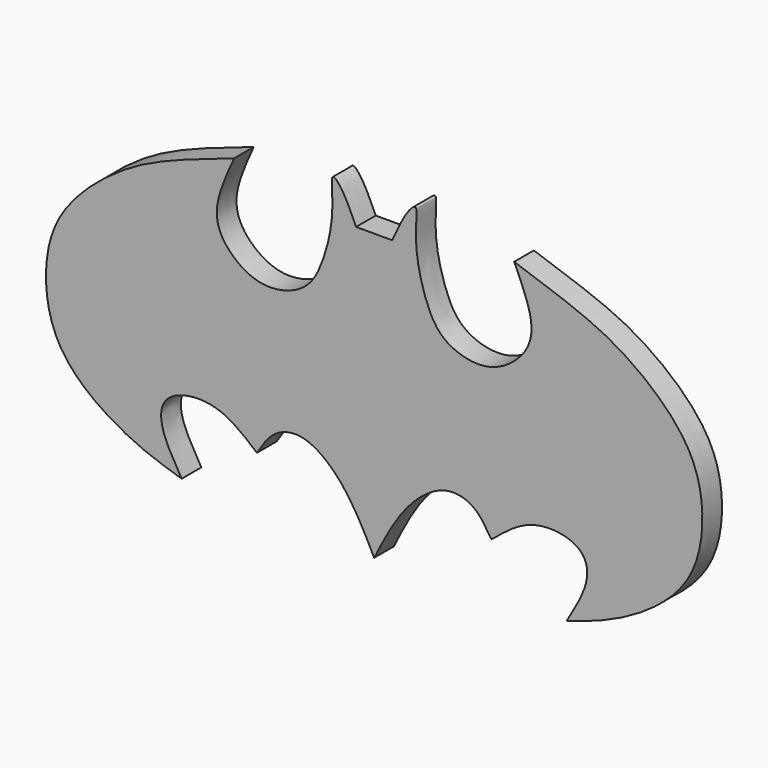
from build123d import *

# Parameters (mm, degrees)
F1_DEPTH = 5


with BuildPart() as f1:
    # F0 (on Front) → F1 (new body)
    with BuildSketch(Plane.XZ):
        with BuildLine():
            Line((-8.2122022286, 40.0784350932), (-11.8819409981, 40.0784350932))
            add(Edge.make_bspline(
                [(-11.8819409981, 40.0784350932), (-12.8782472371, 42.2972484802), (-14.4335544357, 45.7609791067), (-17.3519257227, 48.7913666131), (-16.0950854738, 41.2351091341), (-18.4014485043, 31.4854467346), (-22.0437905993, 24.85808478), (-31.2282103596, 22.4385748293), (-38.4247454255, 27.2876434832), (-41.4317275403, 33.8661623662), (-38.41791048, 40.5091837611), (-36.6988517344, 44.2983135581)],
                knots=[0, 0, 0, 0, 0.1088146702, 0.1698676905, 0.2662726076, 0.4039159487, 0.5157076846, 0.6364836069, 0.7547343235, 0.8601022896, 1, 1, 1, 1], degree=3))
            add(Edge.make_bspline(
                [(-36.6988517344, 44.2983135581), (-40.7675535004, 42.9207700785), (-48.8190673042, 40.1947628707), (-59.720474171, 35.363141512), (-72.7769239422, 24.2824619419), (-75.9139064544, 11.2929836241), (-73.1167440149, -3.1146307179), (-58.8360799137, -12.9740366543), (-50.9861442753, -15.4269461348), (-47.3704449832, -16.5567621589)],
                knots=[0, 0, 0, 0, 0.1374294184, 0.271957721, 0.4283369128, 0.5665488064, 0.709317309, 0.8661108513, 1, 1, 1, 1], degree=3))
            add(Edge.make_bspline(
                [(-47.3704449832, -16.5567621589), (-49.0258540698, -13.767318885), (-51.8526301052, -9.0040664284), (-51.5200005236, -3.7669274307), (-47.3638537079, -1.00085823), (-39.2892684136, -0.8731954731), (-34.5610362718, -4.8462458488), (-32.0631302893, -6.9451923482)],
                knots=[0, 0, 0, 0, 0.2300305605, 0.3928001127, 0.553391391, 0.764058472, 1, 1, 1, 1], degree=3))
            add(Edge.make_bspline(
                [(-32.0631302893, -6.9451923482), (-30.9825657831, -5.1874304781), (-28.8354937584, -1.6947733382), (-22.0931432409, -0.1443481526), (-13.8550388164, -6.7624223585), (-10.1796756768, -14.0692507531), (-8.2122022286, -17.9806984961)],
                knots=[0, 0, 0, 0, 0.2112971318, 0.419845514, 0.689435165, 1, 1, 1, 1], degree=3))
            add(Edge.make_bspline(
                [(15.6387258321, -6.9451923482), (14.5581613259, -5.1874304781), (12.4110893012, -1.6947733382), (5.6687387837, -0.1443481526), (-2.5693656408, -6.7624223585), (-6.2447287804, -14.0692507531), (-8.2122022286, -17.9806984961)],
                knots=[0, 0, 0, 0, 0.2112971318, 0.419845514, 0.689435165, 1, 1, 1, 1], degree=3))
            add(Edge.make_bspline(
                [(30.946040526, -16.5567621589), (32.6014496126, -13.767318885), (35.428225648, -9.0040664284), (35.0955960664, -3.7669274307), (30.9394492507, -1.00085823), (22.8648639564, -0.8731954731), (18.1366318146, -4.8462458488), (15.6387258321, -6.9451923482)],
                knots=[0, 0, 0, 0, 0.2300305605, 0.3928001127, 0.553391391, 0.764058472, 1, 1, 1, 1], degree=3))
            add(Edge.make_bspline(
                [(20.2744472772, 44.2983135581), (24.3431490432, 42.9207700785), (32.394662847, 40.1947628707), (43.2960697138, 35.363141512), (56.352519485, 24.2824619419), (59.4895019971, 11.2929836241), (56.6923395577, -3.1146307179), (42.4116754565, -12.9740366543), (34.5617398181, -15.4269461348), (30.946040526, -16.5567621589)],
                knots=[0, 0, 0, 0, 0.1374294184, 0.271957721, 0.4283369128, 0.5665488064, 0.709317309, 0.8661108513, 1, 1, 1, 1], degree=3))
            add(Edge.make_bspline(
                [(-4.5424634591, 40.0784350932), (-3.5461572201, 42.2972484802), (-1.9908500215, 45.7609791067), (0.9275212655, 48.7913666131), (-0.3293189834, 41.2351091341), (1.9770440471, 31.4854467346), (5.6193861421, 24.85808478), (14.8038059024, 22.4385748293), (22.0003409683, 27.2876434832), (25.0073230831, 33.8661623662), (21.9935060227, 40.5091837611), (20.2744472772, 44.2983135581)],
                knots=[0, 0, 0, 0, 0.1088146702, 0.1698676905, 0.2662726076, 0.4039159487, 0.5157076846, 0.6364836069, 0.7547343235, 0.8601022896, 1, 1, 1, 1], degree=3))
            Line((-4.5424634591, 40.0784350932), (-8.2122022286, 40.0784350932))
        make_face()
        with BuildLine():
            add(Edge.make_bspline(
                [(-40.7788082957, 40.8485867083), (-45.0160925485, 39.1557450069), (-53.0935510599, 35.9287114181), (-62.2941692207, 30.6878977022), (-71.2479782326, 20.5851416615), (-73.0395933906, 13.1368363398), (-70.655821628, 0.3918412405), (-65.9333309108, -4.7486149953), (-56.4205247664, -11.0687593178), (-52.9760592159, -12.4550883248), (-51.5802241862, -13.0168842152)],
                knots=[0, 0, 0, 0, 0.1450786062, 0.2765607292, 0.4190573419, 0.5300860887, 0.6687412322, 0.7763945775, 0.9093861509, 1, 1, 1, 1], degree=3))
            add(Edge.make_bspline(
                [(-12.7671184018, 37.1527262032), (-12.8105221655, 37.767832184), (-12.9167695581, 39.2735404689), (-14.2569275875, 43.199559326), (-15.3833842453, 44.8124103405), (-15.4205368039, 43.5883704744), (-15.2325001114, 42.0644743626), (-15.5858480298, 37.7221519204), (-16.6233242245, 33.2855966544), (-18.8663482525, 24.8126850649), (-23.665219481, 22.8462807986), (-32.7768476073, 20.7730831752), (-39.0865075301, 23.8717377388), (-43.0417250552, 31.6481993654), (-41.5266216034, 37.7005347177), (-40.999533454, 39.9194052312), (-40.7788082957, 40.8485867083)],
                knots=[0, 0, 0, 0, 0.0505373663, 0.1237096266, 0.1629392742, 0.1913954138, 0.2358051509, 0.3063180282, 0.384250961, 0.4831926503, 0.5605011807, 0.6644710974, 0.7540445736, 0.853320775, 0.9385761278, 1, 1, 1, 1], degree=3))
            add(Edge.make_bspline(
                [(-3.9949859492, 37.1527262032), (-6.9190301001, 37.1527262032), (-9.843074251, 37.1527262032), (-12.7671184018, 37.1527262032)],
                knots=[0, 0, 0, 0, 8.7721324526, 8.7721324526, 8.7721324526, 8.7721324526], degree=3))
            add(Edge.make_bspline(
                [(23.7335767597, 41.2493087351), (24.4530114667, 39.9054678233), (26.0244092307, 36.9702346694), (26.4309050247, 30.0518223198), (21.4354728883, 23.0866334692), (16.0479597422, 20.9866016223), (7.9404867152, 21.5334795427), (2.0840254692, 24.9926080902), (-1.1094411846, 32.1097669255), (-2.0201724202, 39.2006909165), (-0.2992768192, 43.7223415812), (-0.8622936336, 45.0976152318), (-1.5127566292, 43.0204295249), (-2.6220619028, 39.8039584717), (-3.553918632, 38.0044644382), (-3.9949859492, 37.1527262032)],
                knots=[0, 0, 0, 0, 0.0759707125, 0.1659361253, 0.2650579009, 0.3479302006, 0.4454920972, 0.5347423734, 0.6305967349, 0.7255041462, 0.8006387765, 0.8294813208, 0.8722005151, 0.9395098257, 1, 1, 1, 1], degree=3))
            add(Edge.make_bspline(
                [(33.6919203401, -14.0843614936), (36.1215948245, -13.1765941813), (40.9033469103, -11.3900510592), (46.9128093998, -7.3858234932), (52.3922477573, -1.9336381195), (55.6792503222, 4.8090224621), (57.3430496625, 14.3121441122), (51.6156153831, 23.3802559022), (46.1096093701, 29.991862224), (34.2840988264, 35.6082745296), (26.8791146652, 39.6051952856), (24.6061054028, 40.7932544385), (23.7335767597, 41.2493087351)],
                knots=[0, 0, 0, 0, 0.0974700928, 0.1918272684, 0.2883916571, 0.3843656764, 0.4907723409, 0.6027746209, 0.7066328683, 0.8340968769, 0.9363156018, 1, 1, 1, 1], degree=3))
            add(Edge.make_bspline(
                [(15.9203130752, -4.4681387953), (17.0357728529, -3.6507396117), (19.5409740796, -1.8149500311), (25.6074769381, 1.673208692), (34.2650515573, 0.1921565778), (38.1250522154, -4.8981844373), (36.9121199249, -10.7908754792), (34.7328056008, -13.0197874016), (33.6919203401, -14.0843614936)],
                knots=[0, 0, 0, 0, 0.1453813722, 0.326510735, 0.5253570285, 0.690702799, 0.8522733072, 1, 1, 1, 1], degree=3))
            add(Edge.make_bspline(
                [(-8.41199141, -15.5372489244), (-7.9095024587, -14.4044748883), (-6.7842766221, -11.8678487411), (-3.7155099659, -6.8588281055), (2.1506322805, -0.0343969426), (8.8089995272, 1.9097644372), (13.6745986257, -0.6725949147), (15.1891981707, -3.2324613465), (15.9203130752, -4.4681387953)],
                knots=[0, 0, 0, 0, 0.1379016266, 0.3088037514, 0.5193421259, 0.6974684541, 0.8539644865, 1, 1, 1, 1], degree=3))
            add(Edge.make_bspline(
                [(-32.7044092119, -4.2089852504), (-31.9543092274, -3.1033377243), (-30.4169220227, -0.8372286791), (-26.6621159645, 2.0828916938), (-19.6879348045, 1.1486292117), (-15.0907003626, -2.8975346703), (-9.8445203676, -10.136611032), (-8.8510687142, -13.8819263464), (-8.41199141, -15.5372489244)],
                knots=[0, 0, 0, 0, 0.1390073425, 0.2849061646, 0.4596494045, 0.6323584219, 0.8375129051, 1, 1, 1, 1], degree=3))
            add(Edge.make_bspline(
                [(-51.5802241862, -13.0168842152), (-51.9566141102, -12.1811170797), (-52.8301859904, -10.241366249), (-54.4122635369, -4.5818082654), (-49.7189754854, -0.077195565), (-43.6358806444, 1.8644629269), (-36.5506154261, -0.1909494177), (-33.9335443794, -2.9249383556), (-32.7044092119, -4.2089852504)],
                knots=[0, 0, 0, 0, 0.1250182086, 0.2901575853, 0.4628741696, 0.6427974632, 0.832236041, 1, 1, 1, 1], degree=3))
        make_face(mode=Mode.SUBTRACT)
        with BuildLine():
            add(Edge.make_bspline(
                [(-12.7671184018, 37.1527262032), (-12.8105221655, 37.767832184), (-12.9167695581, 39.2735404689), (-14.2569275875, 43.199559326), (-15.3833842453, 44.8124103405), (-15.4205368039, 43.5883704744), (-15.2325001114, 42.0644743626), (-15.5858480298, 37.7221519204), (-16.6233242245, 33.2855966544), (-18.8663482525, 24.8126850649), (-23.665219481, 22.8462807986), (-32.7768476073, 20.7730831752), (-39.0865075301, 23.8717377388), (-43.0417250552, 31.6481993654), (-41.5266216034, 37.7005347177), (-40.999533454, 39.9194052312), (-40.7788082957, 40.8485867083)],
                knots=[0, 0, 0, 0, 0.0505373663, 0.1237096266, 0.1629392742, 0.1913954138, 0.2358051509, 0.3063180282, 0.384250961, 0.4831926503, 0.5605011807, 0.6644710974, 0.7540445736, 0.853320775, 0.9385761278, 1, 1, 1, 1], degree=3))
            add(Edge.make_bspline(
                [(-40.7788082957, 40.8485867083), (-45.0160925485, 39.1557450069), (-53.0935510599, 35.9287114181), (-62.2941692207, 30.6878977022), (-71.2479782326, 20.5851416615), (-73.0395933906, 13.1368363398), (-70.655821628, 0.3918412405), (-65.9333309108, -4.7486149953), (-56.4205247664, -11.0687593178), (-52.9760592159, -12.4550883248), (-51.5802241862, -13.0168842152)],
                knots=[0, 0, 0, 0, 0.1450786062, 0.2765607292, 0.4190573419, 0.5300860887, 0.6687412322, 0.7763945775, 0.9093861509, 1, 1, 1, 1], degree=3))
            add(Edge.make_bspline(
                [(-51.5802241862, -13.0168842152), (-51.9566141102, -12.1811170797), (-52.8301859904, -10.241366249), (-54.4122635369, -4.5818082654), (-49.7189754854, -0.077195565), (-43.6358806444, 1.8644629269), (-36.5506154261, -0.1909494177), (-33.9335443794, -2.9249383556), (-32.7044092119, -4.2089852504)],
                knots=[0, 0, 0, 0, 0.1250182086, 0.2901575853, 0.4628741696, 0.6427974632, 0.832236041, 1, 1, 1, 1], degree=3))
            add(Edge.make_bspline(
                [(-32.7044092119, -4.2089852504), (-31.9543092274, -3.1033377243), (-30.4169220227, -0.8372286791), (-26.6621159645, 2.0828916938), (-19.6879348045, 1.1486292117), (-15.0907003626, -2.8975346703), (-9.8445203676, -10.136611032), (-8.8510687142, -13.8819263464), (-8.41199141, -15.5372489244)],
                knots=[0, 0, 0, 0, 0.1390073425, 0.2849061646, 0.4596494045, 0.6323584219, 0.8375129051, 1, 1, 1, 1], degree=3))
            add(Edge.make_bspline(
                [(-8.41199141, -15.5372489244), (-7.9095024587, -14.4044748883), (-6.7842766221, -11.8678487411), (-3.7155099659, -6.8588281055), (2.1506322805, -0.0343969426), (8.8089995272, 1.9097644372), (13.6745986257, -0.6725949147), (15.1891981707, -3.2324613465), (15.9203130752, -4.4681387953)],
                knots=[0, 0, 0, 0, 0.1379016266, 0.3088037514, 0.5193421259, 0.6974684541, 0.8539644865, 1, 1, 1, 1], degree=3))
            add(Edge.make_bspline(
                [(15.9203130752, -4.4681387953), (17.0357728529, -3.6507396117), (19.5409740796, -1.8149500311), (25.6074769381, 1.673208692), (34.2650515573, 0.1921565778), (38.1250522154, -4.8981844373), (36.9121199249, -10.7908754792), (34.7328056008, -13.0197874016), (33.6919203401, -14.0843614936)],
                knots=[0, 0, 0, 0, 0.1453813722, 0.326510735, 0.5253570285, 0.690702799, 0.8522733072, 1, 1, 1, 1], degree=3))
            add(Edge.make_bspline(
                [(33.6919203401, -14.0843614936), (36.1215948245, -13.1765941813), (40.9033469103, -11.3900510592), (46.9128093998, -7.3858234932), (52.3922477573, -1.9336381195), (55.6792503222, 4.8090224621), (57.3430496625, 14.3121441122), (51.6156153831, 23.3802559022), (46.1096093701, 29.991862224), (34.2840988264, 35.6082745296), (26.8791146652, 39.6051952856), (24.6061054028, 40.7932544385), (23.7335767597, 41.2493087351)],
                knots=[0, 0, 0, 0, 0.0974700928, 0.1918272684, 0.2883916571, 0.3843656764, 0.4907723409, 0.6027746209, 0.7066328683, 0.8340968769, 0.9363156018, 1, 1, 1, 1], degree=3))
            add(Edge.make_bspline(
                [(23.7335767597, 41.2493087351), (24.4530114667, 39.9054678233), (26.0244092307, 36.9702346694), (26.4309050247, 30.0518223198), (21.4354728883, 23.0866334692), (16.0479597422, 20.9866016223), (7.9404867152, 21.5334795427), (2.0840254692, 24.9926080902), (-1.1094411846, 32.1097669255), (-2.0201724202, 39.2006909165), (-0.2992768192, 43.7223415812), (-0.8622936336, 45.0976152318), (-1.5127566292, 43.0204295249), (-2.6220619028, 39.8039584717), (-3.553918632, 38.0044644382), (-3.9949859492, 37.1527262032)],
                knots=[0, 0, 0, 0, 0.0759707125, 0.1659361253, 0.2650579009, 0.3479302006, 0.4454920972, 0.5347423734, 0.6305967349, 0.7255041462, 0.8006387765, 0.8294813208, 0.8722005151, 0.9395098257, 1, 1, 1, 1], degree=3))
            add(Edge.make_bspline(
                [(-3.9949859492, 37.1527262032), (-6.9190301001, 37.1527262032), (-9.843074251, 37.1527262032), (-12.7671184018, 37.1527262032)],
                knots=[0, 0, 0, 0, 8.7721324526, 8.7721324526, 8.7721324526, 8.7721324526], degree=3))
        make_face()
    extrude(amount=F1_DEPTH)


solid = f1.part
